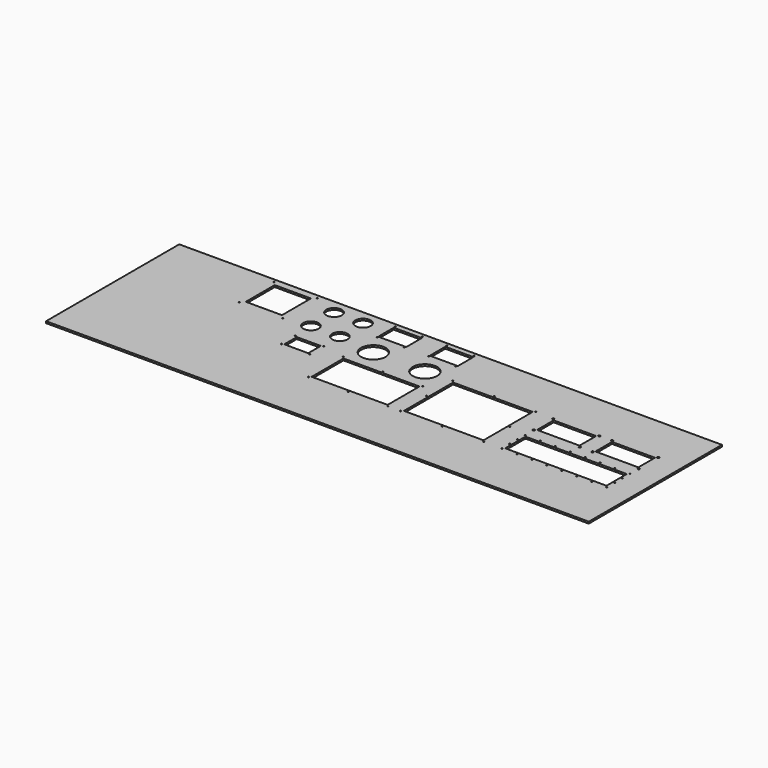
from build123d import *

# Parameters (mm, degrees)
F0_W     = 1905
F0_H     = 584.2
F0_W_2   = 279.4
F0_H_2   = 152.4
F0_W_3   = 368.3
F0_H_3   = 101.6
F0_W_4   = 84.16
F0_H_4   = 55.16
F0_W_5   = 127
F0_H_5   = 127
F0_W_6   = 161.8
F0_H_6   = 85.6
F0_W_7   = 355.6
F0_H_7   = 88.9
F0_H_8   = 215.9
F0_W_8   = 266.7
F0_H_9   = 139.7
F0_W_9   = 149.1
F0_H_10  = 72.9
F0_W_10  = 150.6218942523
F0_W_11  = 95.475
F0_H_11  = 6.35
F0_H_12  = 4.8625
F1_DEPTH = 6.35
F2_D     = 4.1656
F3_D     = 7.0104
F4_D     = 54
F5_D     = 86


# Not quite as in the source:
# - a feature names something its author has since deleted; it is built from what else it names


with BuildPart() as f1:
    # F0 (on Top) → F1 (new body)
    with BuildSketch(Plane.XY):
        with Locations((499.8503303409, 41.4113755345)):
            Rectangle(F0_W, F0_H)
        with Locations((455.4003303409, 16.0113749921)):
            Rectangle(F0_W_2, F0_H_2, mode=Mode.SUBTRACT)
        with Locations((1179.3003303409, -9.3886244655)):
            Rectangle(F0_W_3, F0_H_3, mode=Mode.SUBTRACT)
        with Locations((185.112135537, 77.3313755345)):
            Rectangle(F0_W_4, F0_H_4, mode=Mode.SUBTRACT)
        with Locations((-33.5496696591, 244.6113755345)):
            Rectangle(F0_W_5, F0_H_5, mode=Mode.SUBTRACT)
        Polygon((315.7003303409, 314.4613755345), (315.7003303409, 320.8113755345), (411.1753303409, 320.8113755345), (411.1753303409, 314.4613755345), (414.1253303409, 314.4613755345), (414.1253303409, 246.1988755345), (411.1753303409, 246.1988755345), (411.1753303409, 241.3363755345), (315.7003303409, 241.3363755345), (315.7003303409, 246.1988755345), align=None, mode=Mode.SUBTRACT)
        Polygon((639.5503303409, 54.1113755345), (639.5503303409, 168.4113755345), (931.6503303409, 168.4113755345), (931.6503303409, -60.1886244655), (785.6003303409, -60.1886244655), (639.5503303409, -60.1886244655), align=None, mode=Mode.SUBTRACT)
        with Locations((1076.0503303409, 122.3113755345)):
            Rectangle(F0_W_6, F0_H_6, mode=Mode.SUBTRACT)
        with Locations((1282.5503303409, 122.3113742352)):
            Rectangle(F0_W_6, F0_H_6, mode=Mode.SUBTRACT)
        Polygon((496.6753303409, 314.4613755345), (496.6753303409, 320.8113755345), (592.1503303409, 320.8113755345), (592.1503303409, 314.4613755345), (595.1003303409, 314.4613755345), (595.1003303409, 246.1988755345), (592.1503303409, 246.1988755345), (592.1503303409, 241.3363755345), (496.6753303409, 241.3363755345), (496.6753303409, 246.1988755345), align=None, mode=Mode.SUBTRACT)
        with Locations((1179.3003303409, -9.3886244655)):
            Rectangle(F0_W_3, F0_H_3)
        with Locations((1179.3003303409, -9.3886244655)):
            Rectangle(F0_W_7, F0_H_7, mode=Mode.SUBTRACT)
        Polygon((931.6503303409, 168.4113755345), (639.5503303409, 168.4113755345), (639.5503303409, 54.1113755345), (639.5503303409, -60.1886244655), (785.6003303409, -60.1886244655), (931.6503303409, -60.1886244655), align=None)
        with Locations((785.6003303409, 54.1113755345)):
            Rectangle(F0_W_2, F0_H_8, mode=Mode.SUBTRACT)
        with Locations((455.4003303409, 16.0113749921)):
            Rectangle(F0_W_2, F0_H_2)
        with Locations((455.4003303409, 16.0113749921)):
            Rectangle(F0_W_8, F0_H_9, mode=Mode.SUBTRACT)
        with Locations((1076.0503303409, 122.3113755345)):
            Rectangle(F0_W_6, F0_H_6)
        with Locations((1076.0503303409, 122.3113755345)):
            Rectangle(F0_W_9, F0_H_10, mode=Mode.SUBTRACT)
        with Locations((1282.5503303409, 122.3113742352)):
            Rectangle(F0_W_6, F0_H_6)
        with Locations((1281.7893832147, 122.3113742352)):
            Rectangle(F0_W_10, F0_H_10, mode=Mode.SUBTRACT)
        with Locations((363.4378303409, 317.6363755345)):
            Rectangle(F0_W_11, F0_H_11)
        with Locations((363.4378303409, 243.7676255345)):
            Rectangle(F0_W_11, F0_H_12)
        with Locations((544.4128303409, 317.6363755345)):
            Rectangle(F0_W_11, F0_H_11)
        with Locations((544.4128303409, 243.7676255345)):
            Rectangle(F0_W_11, F0_H_12)
    extrude(amount=F1_DEPTH)

    # F2 (through all)
    with Locations(Plane(origin=(0, 0, 0), x_dir=(1, 0, 0), z_dir=(0, 0, -1))):
        with Locations((995.1503303409, -41.4113755345), (995.1503303409, -7.6293755345), (995.1503303409, 26.1526244655), (995.1503303409, 60.1886244655), (1047.7283303409, 60.1886244655), (1100.3063303409, 60.1886244655), (1152.8843303409, 60.1886244655), (1205.4623303409, 60.1886244655), (1258.0403303409, 60.1886244655), (1310.6183303409, 60.1886244655), (1363.4503303409, 60.1886244655), (1363.4503303409, 26.4066244655), (1363.4503303409, -7.6293755345), (1363.4503303409, -41.4113755345), (1310.6183303409, -41.4113755345), (1258.0403303409, -41.4113755345), (1205.4623303409, -41.4113755345), (1152.8843303409, -41.4113755345), (1100.3063303409, -41.4113755345), (1047.7283303409, -41.4113755345), (639.5503303409, -168.4113755345), (785.6003303409, -168.4113755345), (931.6503303409, -168.4113755345), (931.6503303409, -54.1113755345), (931.6503303409, 60.1886244655), (785.6003303409, 60.1886244655), (639.5503303409, 60.1886244655), (639.5503303409, -54.1113755345), (315.7003303409, -92.2113749921), (455.4003303409, -92.2113749921), (595.1003303409, -92.2113749921), (595.1003303409, 60.1886250079), (455.4003303409, 60.1886250079), (315.7003303409, 60.1886250079), (315.7003303409, -320.8113755345), (411.1753303409, -320.8113755345), (411.1753303409, -241.3363755345), (315.7003303409, -241.3363755345), (496.6753303409, -320.8113755345), (496.6753303409, -241.3363755345), (592.1503303409, -241.3363755345), (592.1503303409, -320.8113755345), (135.614335537, -107.9269755345), (234.614335537, -107.9269755345), (234.614335537, -46.7199755345), (135.614335537, -46.7199755345), (-109.7496696591, -320.8113755345), (-109.7496696591, -168.4113755345), (42.6503303409, -168.4113755345), (42.6503303409, -320.8113755345)):
            Hole(F2_D / 2)

    # F3 (through all)
    with Locations(Plane(origin=(0, 0, 0), x_dir=(1, 0, 0), z_dir=(0, 0, -1))):
        with Locations((995.1503303409, -165.1113755345), (995.1503303409, -79.5113755345), (1156.9503303409, -79.5113755345), (1156.9503303409, -165.1113755345), (1201.6503303409, -165.1113742352), (1201.6503303409, -79.5113742352), (1363.4503303409, -79.5113742352), (1363.4503303409, -165.1113742352)):
            Hole(F3_D / 2)

    # F4 (through all)
    with Locations(Plane(origin=(0, 0, 0), x_dir=(1, 0, 0), z_dir=(0, 0, -1))):
        with Locations((233.1503303409, -181.1113755345), (233.1503303409, -282.7113755345), (131.5503303409, -181.1113755345), (131.5503303409, -282.7113755345)):
            Hole(F4_D / 2)

    # F5 (through all)
    with Locations(Plane(origin=(0, 0, 0), x_dir=(1, 0, 0), z_dir=(0, 0, -1))):
        with Locations((363.4378303409, -165.1363755345), (544.4128303409, -165.1363755345)):
            Hole(F5_D / 2)


solid = f1.part
